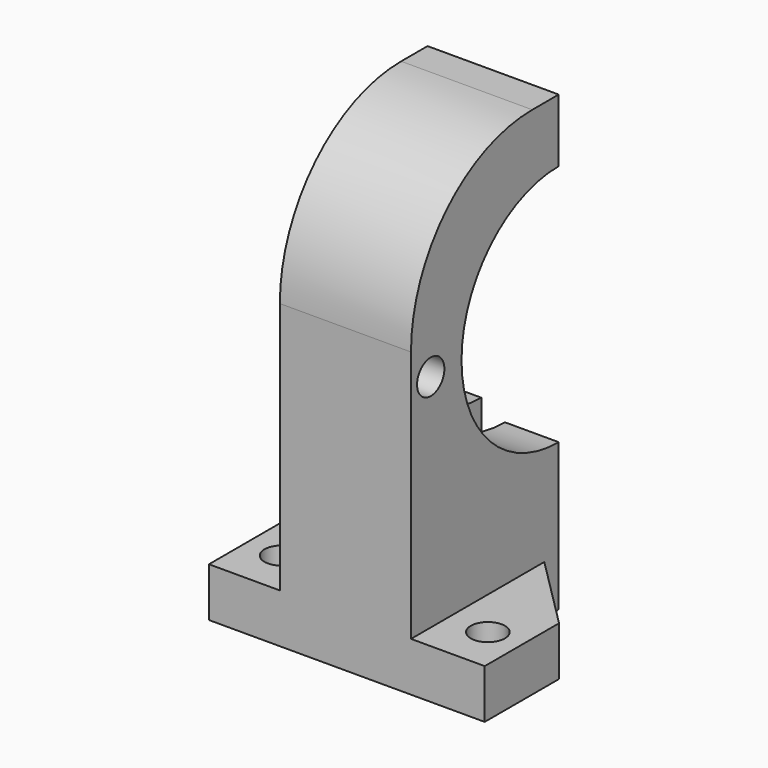
from build123d import *

# Parameters (mm, degrees)
F1_DEPTH     = 5
F3_DEPTH     = 2.2
F5_DEPTH     = 5
F6_R         = 14.1038356314
F7_W         = 8.643694222
F7_H         = 4.569907207
F8_DEPTH     = 6.858
F10_DEPTH    = 25.654
F9_R         = 1.5875
F11_DEPTH    = 26.924
F12_R        = 1.5875
F13_DEPTH    = 9.5758
F14_T4_DEPTH = 4.569907207
F14_T9_DEPTH = 4.569907207
F15_R        = 1.5875
F16_DEPTH    = 18.034


# Not quite as in the source:
# - a fillet or chamfer that OpenCascade refuses, or shapes differently, is made with other operations: its cross-section is extruded or revolved along the edge and cut away or added


with BuildPart() as f1:
    # F0 (on Right) → F1 (new body)
    with BuildSketch(Plane.YZ):
        with BuildLine():
            Line((-17.1746751294, 0), (0, 0))
            Line((0, 0), (0, 15))
            ThreePointArc((0, 15), (-10, 25), (0, 35))
            Line((0, 35), (0, 42.1679355204))
            Line((0, 42.1679355204), (-17.1746751294, 42.1679355204))
            Line((-17.1746751294, 42.1679355204), (-17.1746751294, 0))
        make_face()
    extrude(amount=F1_DEPTH)

    # F2 (on face) → F3 (join)
    with BuildSketch(Plane.YZ.offset(5)):
        with BuildLine():
            ThreePointArc((0, 10.8), (-14.2, 25), (0, 39.2))
            Line((0, 39.2), (0, 42.1679355204))
            Line((0, 42.1679355204), (-17.1746751294, 42.1679355204))
            Line((-17.1746751294, 42.1679355204), (-17.1746751294, 0))
            Line((-17.1746751294, 0), (0, 0))
            Line((0, 0), (0, 10.8))
        make_face()
    extrude(amount=F3_DEPTH)

    # F4 (on face) → F5 (join)
    with BuildSketch(Plane.YZ.offset(7.2)):
        with BuildLine():
            ThreePointArc((0, 10.8), (-14.2, 25), (0, 39.2))
            Line((0, 39.2), (0, 42.1679355204))
            Line((0, 42.1679355204), (-17.1746751294, 42.1679355204))
            Line((-17.1746751294, 42.1679355204), (-17.1746751294, 0))
            Line((-17.1746751294, 0), (0, 0))
            Line((0, 0), (0, 10.8))
        make_face()
        with BuildLine():
            ThreePointArc((0, 13.7), (-11.3, 25), (0, 36.3))
            Line((0, 36.3), (0, 39.2))
            ThreePointArc((0, 39.2), (-14.2, 25), (0, 10.8))
            Line((0, 10.8), (0, 13.7))
        make_face()
    extrude(amount=F5_DEPTH)

    # F6
    f6_edges = [f1.edges().sort_by_distance(p)[0] for p in [
        (6.1, -17.174675, 42.167936),
    ]]
    fillet(f6_edges, radius=F6_R)

    # F7 (on face) → F8 (join)
    with BuildSketch(Plane.YZ.offset(12.2)):
        with Locations((-12.8528280184, 2.2849536035)):
            Rectangle(F7_W, F7_H)
    extrude(amount=F8_DEPTH)

    # F10 (add): a face of the model
    f10_faces = [f1.faces().sort_by_distance(p)[0] for p in [
        (19.058, -12.8528280184, 2.2849536035),
    ]]
    extrude(f10_faces, amount=-F10_DEPTH)

    # F9 (on face) → F11 (cut)
    with BuildSketch(Plane.XY.offset(4.569907207)):
        with Locations((15.894247219, -12.8528280184)):
            Circle(F9_R)
    extrude(amount=-F11_DEPTH, mode=Mode.SUBTRACT)

    # F12 (on face) → F13 (cut)
    with BuildSketch(Plane.XY.offset(4.569907207)):
        with Locations((-3.329155501, -12.8116961569)):
            Circle(F12_R)
    extrude(amount=-F13_DEPTH, mode=Mode.SUBTRACT)

    # F14: chamfer of 6.858 on 2 edges, made by hand


with BuildPart() as f14_tool2:
    # F14_s3 → F14_t4 (new body)
    with BuildSketch(Plane.XY):
        Polygon((12.2, -1.6729809074), (19.058, -8.5309809074), (12.2, -8.5309809074), align=None)
    extrude(amount=F14_T4_DEPTH)

    split(bisect_by=Plane.YZ.offset(19.058), keep=Keep.BOTTOM)


with BuildPart() as f1_1:
    add(f1.part)

    # F14_t1: union F14_tool2
    add(f14_tool2.part)


with BuildPart() as f14_tool7:
    # F14_s8 → F14_t9 (new body)
    with BuildSketch(Plane.XY):
        Polygon((0, -1.6729809074), (-6.858, -8.5309809074), (0, -8.5309809074), align=None)
    extrude(amount=F14_T9_DEPTH)

    split(bisect_by=Plane.YZ.offset(-6.596), keep=Keep.TOP)


with BuildPart() as f1_2:
    add(f1_1.part)

    # F14_t6: union F14_tool7
    add(f14_tool7.part)

    # F15 (on face) → F16 (cut)
    with BuildSketch(Plane.YZ.offset(12.2)):
        with Locations((-14.881552197, 25.1055490226)):
            Circle(F15_R)
    extrude(amount=-F16_DEPTH, mode=Mode.SUBTRACT)


solid = f1_2.part
